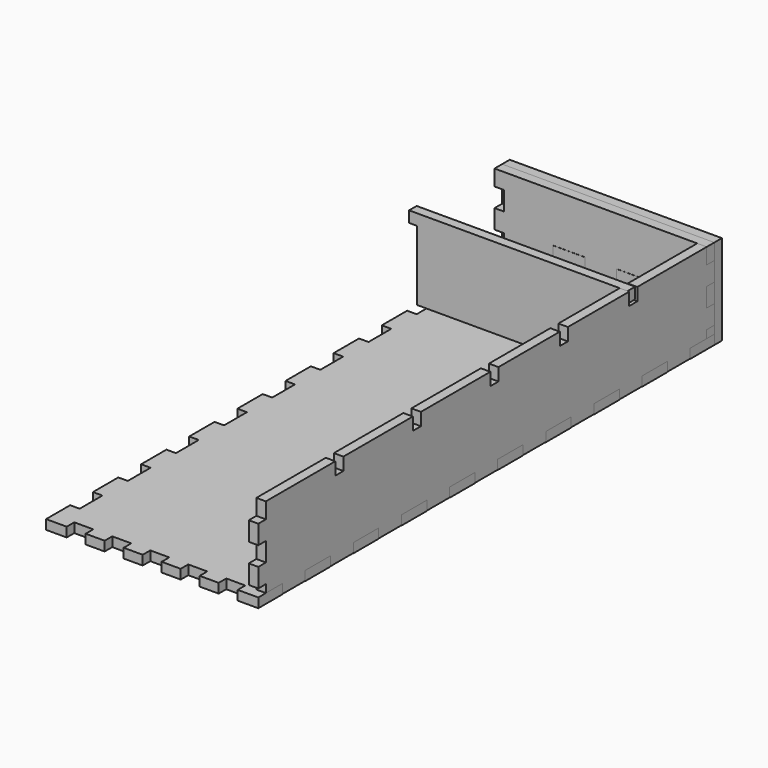
from build123d import *

# Parameters (mm, degrees)
F0_W      = 10
F0_H      = 3.0292458832
F0_W_2    = 3
F0_H_2    = 6
F1_DEPTH  = 3
F3_DEPTH  = 3
F4_W      = 9
F4_H      = 2.9129978023
F4_W_2    = 3
F4_H_2    = 6
F5_DEPTH  = 3
F6_W      = 10
F6_H      = 3
F7_DEPTH  = 3
F9_W      = 3.2
F9_H      = 4
F10_DEPTH = 67.001
F11_W     = 2.5
F11_H     = 3.5
F12_DEPTH = 3
F8_W      = 3
F8_H      = 6
F8_W_2    = 6.5
F8_H_2    = 3
F8_W_3    = 6
F13_DEPTH = 3


with BuildPart() as f1:
    # F0 (on Front) → F1 (new body)
    with BuildSketch(Plane.XZ):
        Polygon((6.5, 3), (6.5, 0), (12.5, 0), (12.5, 3), (18.5, 3), (18.5, 0), (24.5, 0), (24.5, 3), (30.5, 3), (30.5, 0), (36.5, 0), (36.5, 3), (42.5, 3), (42.5, 0), (48.5, 0), (48.5, 3), (54.5, 3), (54.5, 0), (60.5, 0), (60.5, 3), (67, 3), (67, 5.5), (64, 5.5), (64, 11.5), (64, 17.5), (64, 23.5), (67, 23.5), (67, 28.5), (0, 28.5), (0, 23.5), (3, 23.5), (3, 17.5), (3, 11.5), (3, 5.5), (0, 5.5), (0, 3), align=None)
        with Locations((23.5, 11.6221904755)):
            Rectangle(F0_W, F0_H, mode=Mode.SUBTRACT)
        with Locations((43.5, 11.6221904755)):
            Rectangle(F0_W, F0_H, mode=Mode.SUBTRACT)
        with Locations((1.5, 14.5)):
            Rectangle(F0_W_2, F0_H_2)
        with Locations((65.5, 14.5)):
            Rectangle(F0_W_2, F0_H_2)
    extrude(amount=F1_DEPTH)


with BuildPart() as f3:
    # F2 (on Top) → F3 (new body)
    with BuildSketch(Plane.XY):
        Polygon((0, -170.5), (0, -180), (6.5, -180), (6.5, -177), (12.5, -177), (12.5, -180), (18.5, -180), (18.5, -177), (24.5, -177), (24.5, -180), (30.5, -180), (30.5, -177), (36.5, -177), (36.5, -180), (42.5, -180), (42.5, -177), (48.5, -177), (48.5, -180), (54.5, -180), (54.5, -177), (60.5, -177), (60.5, -180), (67, -180), (67, -170.5), (64, -170.5), (64, -161.5), (67, -161.5), (67, -151.5), (64, -151.5), (64, -142.5), (67, -142.5), (67, -132.5), (64, -132.5), (64, -123.5), (67, -123.5), (67, -113.5), (64, -113.5), (64, -104.5), (67, -104.5), (67, -94.5), (64, -94.5), (64, -85.5), (67, -85.5), (67, -75.5), (64, -75.5), (64, -66.5), (67, -66.5), (67, -56.5), (64, -56.5), (64, -47.5), (67, -47.5), (67, -37.5), (64, -37.5), (64, -28.5), (67, -28.5), (67, -18.5), (64, -18.5), (64, -9.5), (67, -9.5), (67, 0), (60.5, 0), (60.5, -3), (54.5, -3), (54.5, 0), (48.5, 0), (48.5, -3), (42.5, -3), (42.5, 0), (36.5, 0), (36.5, -3), (30.5, -3), (30.5, 0), (24.5, 0), (24.5, -3), (18.5, -3), (18.5, 0), (12.5, 0), (12.5, -3), (6.5, -3), (6.5, 0), (0, 0), (0, -9.5), (3, -9.5), (3, -18.5), (0, -18.5), (0, -28.5), (3, -28.5), (3, -37.5), (0, -37.5), (0, -47.5), (3, -47.5), (3, -56.5), (0, -56.5), (0, -66.5), (3, -66.5), (3, -75.5), (0, -75.5), (0, -85.5), (3, -85.5), (3, -94.5), (0, -94.5), (0, -104.5), (3, -104.5), (3, -113.5), (0, -113.5), (0, -123.5), (3, -123.5), (3, -132.5), (0, -132.5), (0, -142.5), (3, -142.5), (3, -151.5), (0, -151.5), (0, -161.5), (3, -161.5), (3, -170.5), align=None)
    extrude(amount=F3_DEPTH)


with BuildPart() as f5:
    # F4 (on face) → F5 (new body)
    with BuildSketch(Plane.YZ.offset(67)):
        Polygon((-28.5, 3), (-18.5, 3), (-9.5, 3), (-3, 3), (-3, 5.5), (-3, 11.5), (-3, 17.5), (-3, 23.5), (-3, 28.5), (-177, 28.5), (-177, 23.5), (-177, 17.5), (-177, 11.5), (-177, 5.5), (-177, 3), (-170.5, 3), (-161.5, 3), (-151.5, 3), (-142.5, 3), (-132.5, 3), (-123.5, 3), (-113.5, 3), (-104.5, 3), (-94.5, 3), (-85.5, 3), (-75.5, 3), (-66.5, 3), (-56.5, 3), (-47.5, 3), (-37.5, 3), align=None)
        with Locations((-166, 1.5435010988)):
            Rectangle(F4_W, F4_H)
        with Locations((-147, 1.5435010988)):
            Rectangle(F4_W, F4_H)
        with Locations((-128, 1.5435010988)):
            Rectangle(F4_W, F4_H)
        with Locations((-109, 1.5435010988)):
            Rectangle(F4_W, F4_H)
        with Locations((-90, 1.5435010988)):
            Rectangle(F4_W, F4_H)
        with Locations((-71, 1.5435010988)):
            Rectangle(F4_W, F4_H)
        with Locations((-52, 1.5435010988)):
            Rectangle(F4_W, F4_H)
        with Locations((-33, 1.5435010988)):
            Rectangle(F4_W, F4_H)
        with Locations((-14, 1.5435010988)):
            Rectangle(F4_W, F4_H)
        with Locations((-1.5, 8.5)):
            Rectangle(F4_W_2, F4_H_2)
        with Locations((-1.5, 20.5)):
            Rectangle(F4_W_2, F4_H_2)
        with Locations((-178.5, 8.5)):
            Rectangle(F4_W_2, F4_H_2)
        with Locations((-178.5, 20.5)):
            Rectangle(F4_W_2, F4_H_2)
    extrude(amount=-F5_DEPTH)

    # F9 (on face) → F10 (cut, through all)
    with BuildSketch(Plane.YZ.offset(67)):
        with Locations((-148, 26.5)):
            Rectangle(F9_W, F9_H)
        with Locations((-117.4, 26.5)):
            Rectangle(F9_W, F9_H)
        with Locations((-86.8, 26.5)):
            Rectangle(F9_W, F9_H)
        with Locations((-59.4, 26.5)):
            Rectangle(F9_W, F9_H)
        with Locations((-32, 26.5)):
            Rectangle(F9_W, F9_H)
    extrude(amount=-F10_DEPTH, mode=Mode.SUBTRACT)


with BuildPart() as f7:
    # F6 (on face) → F7 (new body)
    with BuildSketch(Plane.XY.offset(10.1075675339)):
        with BuildLine():
            Line((48.5, 0), (58.5, 0))
            Line((58.5, 0), (58.5, 5))
            ThreePointArc((58.5, 5), (55.5710678119, 12.0710678119), (48.5, 15))
            Line((48.5, 15), (18.5, 15))
            ThreePointArc((18.5, 15), (11.4289321881, 12.0710678119), (8.5, 5))
            Line((8.5, 5), (8.5, 0))
            Line((8.5, 0), (18.5, 0))
            Line((18.5, 0), (28.5, 0))
            Line((28.5, 0), (38.5, 0))
            Line((38.5, 0), (48.5, 0))
        make_face()
        with Locations((23.5, -1.5)):
            Rectangle(F6_W, F6_H)
        with Locations((43.5, -1.5)):
            Rectangle(F6_W, F6_H)
    extrude(amount=F7_DEPTH)


with BuildPart() as f12:
    # F11 (on face) → F12 (new body)
    with BuildSketch(Plane(origin=(0, -33.6, 0), x_dir=(-1, 0, 0), z_dir=(0, 1, 0))):
        Polygon((0, 28.5), (-64, 28.5), (-64, 25), (-64, 24.5), (-64, 3), (0, 3), (0, 24.5), (0, 25), align=None)
        with Locations((1.25, 26.75)):
            Rectangle(F11_W, F11_H)
        with Locations((-65.25, 26.75)):
            Rectangle(F11_W, F11_H)
    extrude(amount=F12_DEPTH)


with BuildPart() as f13:
    # F8 (on face) → F13 (new body)
    with BuildSketch(Plane(origin=(0, 0, 0), x_dir=(-1, 0, 0), z_dir=(0, 1, 0))):
        Polygon((0, 23.5), (0, 28.5), (-67, 28.5), (-67, 23.5), (-64, 23.5), (-64, 17.5), (-67, 17.5), (-67, 11.5), (-64, 11.5), (-64, 5.5), (-67, 5.5), (-67, 3), (-60.5, 3), (-60.5, 0), (-54.5, 0), (-54.5, 3), (-48.5, 3), (-48.5, 0), (-42.5, 0), (-42.5, 3), (-36.5, 3), (-36.5, 0), (-30.5, 0), (-30.5, 3), (-24.5, 3), (-24.5, 0), (-18.5, 0), (-18.5, 3), (-12.5, 3), (-12.5, 0), (-6.5, 0), (-6.5, 3), (0, 3), (0, 5.5), (-3, 5.5), (-3, 11.5), (0, 11.5), (0, 17.5), (-3, 17.5), (-3, 23.5), align=None)
        Polygon((-38.5, 10.1075675339), (-48.5, 10.1075675339), (-58.5, 10.1075675339), (-58.5, 13.1075675339), (-48.5, 13.1075675339), (-48.5, 13.1368134171), (-38.5, 13.1368134171), (-38.5, 13.1075675339), (-28.5, 13.1075675339), (-28.5, 13.1368134171), (-18.5, 13.1368134171), (-18.5, 13.1075675339), (-8.5, 13.1075675339), (-8.5, 10.1075675339), (-18.5, 10.1075675339), (-28.5, 10.1075675339), align=None, mode=Mode.SUBTRACT)
        with Locations((-1.5, 20.5)):
            Rectangle(F8_W, F8_H)
        with Locations((-65.5, 20.5)):
            Rectangle(F8_W, F8_H)
        with Locations((-1.5, 8.5)):
            Rectangle(F8_W, F8_H)
        with Locations((-65.5, 8.5)):
            Rectangle(F8_W, F8_H)
        with Locations((-3.25, 1.5)):
            Rectangle(F8_W_2, F8_H_2)
        with Locations((-63.75, 1.5)):
            Rectangle(F8_W_2, F8_H_2)
        with Locations((-15.5, 1.5)):
            Rectangle(F8_W_3, F8_H_2)
        with Locations((-51.5, 1.5)):
            Rectangle(F8_W_3, F8_H_2)
        with Locations((-27.5, 1.5)):
            Rectangle(F8_W_3, F8_H_2)
        with Locations((-39.5, 1.5)):
            Rectangle(F8_W_3, F8_H_2)
    extrude(amount=F13_DEPTH)


solid = Compound([f1.part, f3.part, f5.part, f7.part, f12.part, f13.part])
